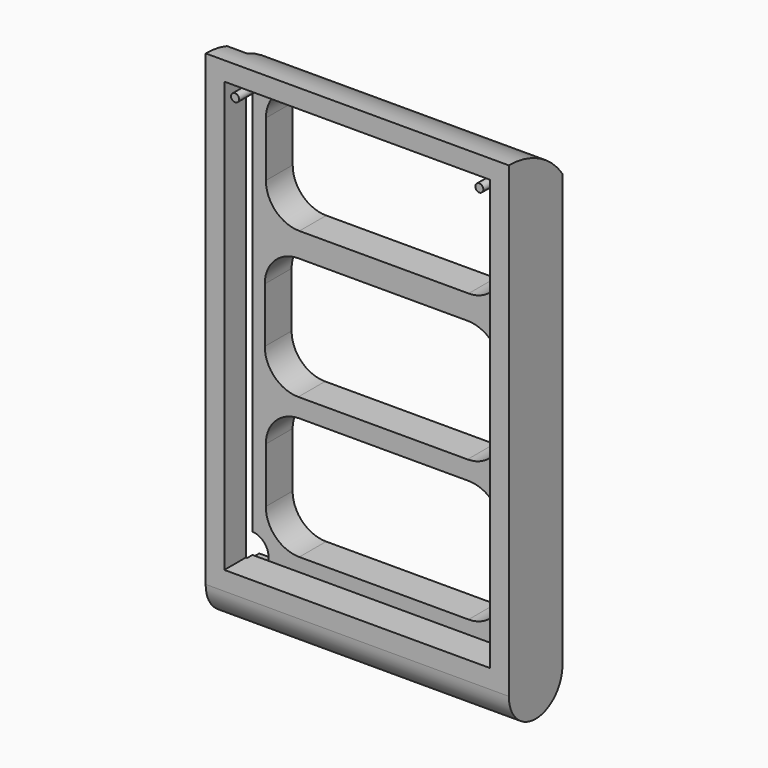
from build123d import *

# Parameters (mm, degrees)
F0_W      = 57.4675095904
F0_H      = 88.5825127872
F1_DEPTH  = 12.7
F3_DEPTH  = 57.4685095904
F4_W      = 50.3555086569
F4_H      = 81.4705118537
F5_DEPTH  = 6.35
F6_R      = 0.7619995332
F8_DEPTH  = 6.35
F11_DEPTH = 56.388
F12_DEPTH = 1.0668
F15_DEPTH = 6.35
F16_DEPTH = 3.81


# Not quite as in the source:
# - a feature of the source that left no trace in its solid (it failed there, or was rolled back) is left out


with BuildPart() as f1:
    # F0 (on Front) → F1 (new body)
    with BuildSketch(Plane.XZ):
        with Locations((8.6671997911, 9.8971910775)):
            Rectangle(F0_W, F0_H)
        with BuildLine():
            ThreePointArc((-13.7333380541, -11.5169252571), (-11.8734661146, -7.0267971965), (-7.3833380541, -5.1669252571))
            Line((-7.3833380541, -5.1669252571), (24.6841715364, -5.1669252571))
            ThreePointArc((24.6841715364, -5.1669252571), (29.1742995969, -7.0267971965), (31.0341715364, -11.5169252571))
            Line((31.0341715364, -11.5169252571), (31.0341715364, -21.9464536455))
            ThreePointArc((31.0341715364, -21.9464536455), (29.1742995969, -26.436581706), (24.6841715364, -28.2964536455))
            Line((24.6841715364, -28.2964536455), (-7.3833380541, -28.2964536455))
            ThreePointArc((-7.3833380541, -28.2964536455), (-11.8734661146, -26.436581706), (-13.7333380541, -21.9464536455))
            Line((-13.7333380541, -21.9464536455), (-13.7333380541, -11.5169252571))
        make_face(mode=Mode.SUBTRACT)
        with BuildLine():
            ThreePointArc((-13.9270129099, 15.1340997942), (-12.0671409704, 19.6242278547), (-7.5770129099, 21.4840997942))
            Line((-7.5770129099, 21.4840997942), (24.4904966805, 21.4840997942))
            ThreePointArc((24.4904966805, 21.4840997942), (28.980624741, 19.6242278547), (30.8404966805, 15.1340997942))
            Line((30.8404966805, 15.1340997942), (30.8404966805, 4.7045714058))
            ThreePointArc((30.8404966805, 4.7045714058), (28.980624741, 0.2144433453), (24.4904966805, -1.6454285942))
            Line((24.4904966805, -1.6454285942), (-7.5770129099, -1.6454285942))
            ThreePointArc((-7.5770129099, -1.6454285942), (-12.0671409704, 0.2144433453), (-13.9270129099, 4.7045714058))
            Line((-13.9270129099, 4.7045714058), (-13.9270129099, 15.1340997942))
        make_face(mode=Mode.SUBTRACT)
        with BuildLine():
            ThreePointArc((-13.7165550041, 42.8851837456), (-11.8566830647, 47.3753118062), (-7.3665550041, 49.2351837456))
            Line((-7.3665550041, 49.2351837456), (24.7009545863, 49.2351837456))
            ThreePointArc((24.7009545863, 49.2351837456), (29.1910826468, 47.3753118062), (31.0509545863, 42.8851837456))
            Line((31.0509545863, 42.8851837456), (31.0509545863, 32.4556553572))
            ThreePointArc((31.0509545863, 32.4556553572), (29.1910826468, 27.9655272967), (24.7009545863, 26.1056553572))
            Line((24.7009545863, 26.1056553572), (-7.3665550041, 26.1056553572))
            ThreePointArc((-7.3665550041, 26.1056553572), (-11.8566830647, 27.9655272967), (-13.7165550041, 32.4556553572))
            Line((-13.7165550041, 32.4556553572), (-13.7165550041, 42.8851837456))
        make_face(mode=Mode.SUBTRACT)
    extrude(amount=F1_DEPTH)

    # F2 (on face) → F3 (cut, through all)
    with BuildSketch(Plane.YZ.offset(37.4009545863)):
        with BuildLine():
            ThreePointArc((-12.7, 54.1884474711), (-5.5566722855, 52.456369837), (0, 47.6448610425))
            Line((0, 47.6448610425), (0, 54.1884474711))
            Line((0, 54.1884474711), (-12.7, 54.1884474711))
        make_face()
    extrude(amount=-F3_DEPTH, mode=Mode.SUBTRACT)

    # F4 (on face) → F5 (cut)
    with BuildSketch(Plane.XZ.offset(12.7)):
        with Locations((8.6671997911, 9.8971910775)):
            Rectangle(F4_W, F4_H)
        with BuildLine():
            Line((-13.7333380541, -21.9464536455), (-13.7333380541, -11.5169252571))
            ThreePointArc((-13.7333380541, -11.5169252571), (-11.8734661146, -7.0267971965), (-7.3833380541, -5.1669252571))
            Line((-7.3833380541, -5.1669252571), (24.6841715364, -5.1669252571))
            ThreePointArc((24.6841715364, -5.1669252571), (29.1742995969, -7.0267971965), (31.0341715364, -11.5169252571))
            Line((31.0341715364, -11.5169252571), (31.0341715364, -21.9464536455))
            ThreePointArc((31.0341715364, -21.9464536455), (29.1742995969, -26.436581706), (24.6841715364, -28.2964536455))
            Line((24.6841715364, -28.2964536455), (-7.3833380541, -28.2964536455))
            ThreePointArc((-7.3833380541, -28.2964536455), (-11.8734661146, -26.436581706), (-13.7333380541, -21.9464536455))
        make_face(mode=Mode.SUBTRACT)
        with BuildLine():
            Line((24.4904966805, -1.6454285942), (-7.5770129099, -1.6454285942))
            ThreePointArc((-7.5770129099, -1.6454285942), (-12.0671409704, 0.2144433453), (-13.9270129099, 4.7045714058))
            Line((-13.9270129099, 4.7045714058), (-13.9270129099, 15.1340997942))
            ThreePointArc((-13.9270129099, 15.1340997942), (-12.0671409704, 19.6242278547), (-7.5770129099, 21.4840997942))
            Line((-7.5770129099, 21.4840997942), (24.4904966805, 21.4840997942))
            ThreePointArc((24.4904966805, 21.4840997942), (28.980624741, 19.6242278547), (30.8404966805, 15.1340997942))
            Line((30.8404966805, 15.1340997942), (30.8404966805, 4.7045714058))
            ThreePointArc((30.8404966805, 4.7045714058), (28.980624741, 0.2144433453), (24.4904966805, -1.6454285942))
        make_face(mode=Mode.SUBTRACT)
        with BuildLine():
            ThreePointArc((-7.3665550041, 26.1056553572), (-11.8566830647, 27.9655272967), (-13.7165550041, 32.4556553572))
            Line((-13.7165550041, 32.4556553572), (-13.7165550041, 42.8851837456))
            ThreePointArc((-13.7165550041, 42.8851837456), (-11.8566830647, 47.3753118062), (-7.3665550041, 49.2351837456))
            Line((-7.3665550041, 49.2351837456), (24.7009545863, 49.2351837456))
            ThreePointArc((24.7009545863, 49.2351837456), (29.1910826468, 47.3753118062), (31.0509545863, 42.8851837456))
            Line((31.0509545863, 42.8851837456), (31.0509545863, 32.4556553572))
            ThreePointArc((31.0509545863, 32.4556553572), (29.1910826468, 27.9655272967), (24.7009545863, 26.1056553572))
            Line((24.7009545863, 26.1056553572), (-7.3665550041, 26.1056553572))
        make_face(mode=Mode.SUBTRACT)
    extrude(amount=-F5_DEPTH, mode=Mode.SUBTRACT)

    # F6 (on face) → F8 (join)
    with BuildSketch(Plane.XZ.offset(6.35)):
        with Locations((-14.4785545374, 48.6004470043)):
            Circle(F6_R)
        with Locations((31.8129541195, 48.6004470043)):
            Circle(F6_R)
    extrude(amount=F8_DEPTH)

    # F10 (on face) → F11 (join)
    with BuildSketch(Plane.YZ.offset(37.4009545863)):
        with BuildLine():
            Line((0, -34.3940653161), (-12.7, -34.3940653161))
            ThreePointArc((-12.7, -34.3940653161), (-6.35, -40.7440653161), (0, -34.3940653161))
        make_face()
    extrude(amount=-F11_DEPTH)

    # F12 (add): a face of the model
    f12_faces = [f1.faces().sort_by_distance(p)[0] for p in [
        (-18.9870454137, -6.35, -37.0890890192),
    ]]
    extrude(f12_faces, amount=F12_DEPTH)

    # F14 (on face) → F15 (cut)
    with BuildSketch(Plane(origin=(0, 0, 0), x_dir=(-1, 0, 0), z_dir=(0, 1, 0))):
        with BuildLine():
            Line((16.464073211, -26.9519573744), (16.464073211, -33.4652290945))
            ThreePointArc((16.464073211, -33.4652290945), (18.7668625115, -32.5113825349), (19.720709071, -30.2085932344))
            ThreePointArc((19.720709071, -30.2085932344), (18.7668625115, -27.9058039339), (16.464073211, -26.9519573744))
        make_face()
        with BuildLine():
            ThreePointArc((16.464073211, -26.9519573744), (13.2074373509, -30.2085932344), (16.464073211, -33.4652290945))
            Line((16.464073211, -33.4652290945), (16.464073211, -26.9519573744))
        make_face()
    extrude(amount=-F15_DEPTH, mode=Mode.SUBTRACT)

    # F13 (on face) → F16 (cut)
    with BuildSketch(Plane(origin=(-20.0665550041, 0, 0), x_dir=(0, -1, 0), z_dir=(-1, 0, 0))):
        with BuildLine():
            Line((0, -34.3940653161), (7.6183550991, -34.3940653161))
            Line((7.6183550991, -34.3940653161), (7.6183550991, 53.3373526242))
            ThreePointArc((7.6183550991, 53.3373526242), (3.3646993114, 51.0859593692), (0, 47.6448610425))
            Line((0, 47.6448610425), (0, -34.3940653161))
        make_face()
    extrude(amount=-F16_DEPTH, mode=Mode.SUBTRACT)


solid = f1.part
